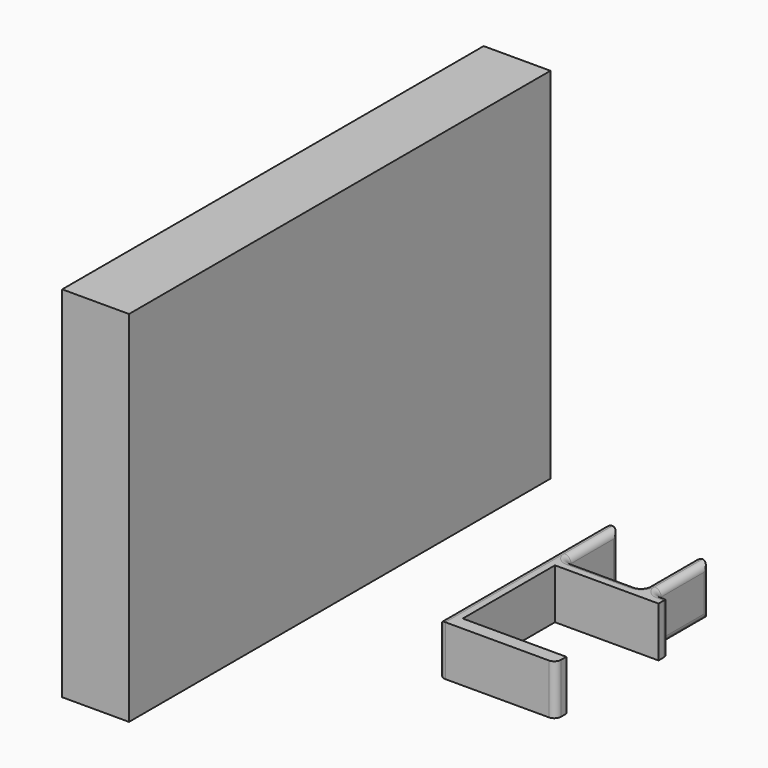
from build123d import *

# Parameters (mm, degrees)
F0_W     = 20
F0_H     = 157.6981320977
F1_DEPTH = 7.5
F0_W_2   = 4
F0_H_2   = 20
F2_R     = 1.99999
F3_DEPTH = 100


# Not quite as in the source:
# - a fillet or chamfer is up to 0.001 mm smaller than in the source, because OpenCascade refuses the exact size


with BuildPart() as f1:
    # F0 (on Top) → F1 (new body, symmetric)
    with BuildSketch(Plane.XY):
        with Locations((-57.7521377802, -12.2206695378)):
            Rectangle(F0_W, F0_H)
    extrude(amount=F1_DEPTH, both=True)

    # F0 (on Top) → F3 (join)
    with BuildSketch(Plane.XY):
        with Locations((-57.7521377802, -12.2206695378)):
            Rectangle(F0_W, F0_H)
    extrude(amount=F3_DEPTH)


with BuildPart() as f1b:
    # F0 (on Top) → F1, piece 2 (new body, symmetric)
    with BuildSketch(Plane.XY):
        with Locations((23.4704200836, 24.5355388032)):
            Rectangle(F0_W_2, F0_H_2)
        Polygon((29.4704200836, 10.5355388032), (29.4704200836, 14.5355388032), (25.4704200836, 14.5355388032), (21.4704200836, 14.5355388032), (-1.5295799164, 14.5355388032), (-5.5295799164, 14.5355388032), (-5.5295799164, -27.9644611968), (29.4704200836, -27.9644611968), (29.4704200836, -23.9644611968), (27.4704200836, -23.9644611968), (-1.5295799164, -23.9644611968), (-1.5295799164, 10.5355388032), (27.4704200836, 10.5355388032), align=None)
        with Locations((-3.5295799164, 24.5355388032)):
            Rectangle(F0_W_2, F0_H_2)
    extrude(amount=F1_DEPTH, both=True)

    # F2 (radius 2 in the source; OpenCascade refuses exactly that, so slightly less here)
    f2_edges = [f1b.edges().sort_by_distance(p)[0] for p in [
        (9.97042, 14.535539, 7.5),
        (27.47042, 14.535539, 7.5),
        (9.97042, 14.535539, -7.5),
        (27.47042, 14.535539, -7.5),
        (-5.52958, 3.285539, 7.5),
        (29.47042, -27.964461, 0),
        (-5.52958, -27.964461, 0),
        (29.47042, 14.535539, 0),
        (25.47042, 34.535539, 0),
        (-1.52958, 34.535539, 0),
        (21.47042, 34.535539, 0),
        (-5.52958, 34.535539, 0),
        (25.47042, 14.535539, 0),
        (21.47042, 14.535539, 0),
        (-1.52958, 14.535539, 0),
        (25.47042, 24.535539, -7.5),
        (25.47042, 24.535539, 7.5),
        (-1.52958, 24.535539, -7.5),
        (-1.52958, 24.535539, 7.5),
        (21.47042, 24.535539, -7.5),
        (21.47042, 24.535539, 7.5),
    ]]
    fillet(f2_edges, radius=F2_R)


solid = Compound([f1.part, f1b.part])
